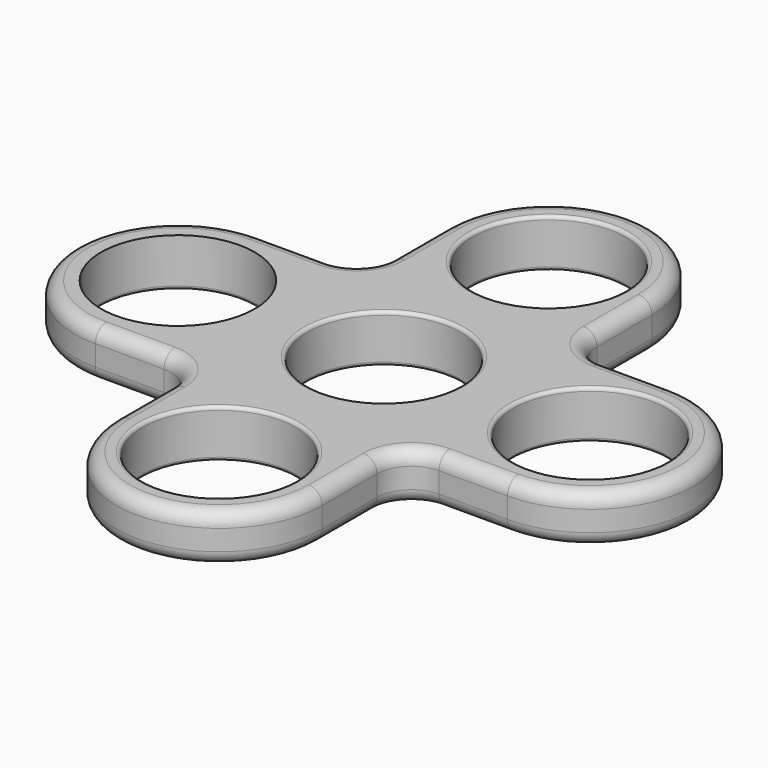
from build123d import *

# Parameters (mm, degrees)
F0_R     = 11.175
F1_DEPTH = 7
F2_R     = 5
F3_R     = 0.5
F4_R     = 2


# Not quite as in the source:
# - a feature names something its author has since deleted; it is built from what else it names


with BuildPart() as f1:
    # F0 (on Top) → F1 (new body)
    with BuildSketch(Plane.XY):
        with BuildLine():
            ThreePointArc((0.5794421554, 15.011195952), (10.8095243265, 19.6002796271), (15, 30))
            ThreePointArc((15, 30), (0, 45), (-15, 30))
            ThreePointArc((-15, 30), (-10.8095243265, 19.6002796271), (-0.5794421554, 15.011195952))
            Line((-0.5794421554, 15.011195952), (-0.011195952, 15.011195952))
            Line((-0.011195952, 15.011195952), (0.011195952, 15.011195952))
            Line((0.011195952, 15.011195952), (0.5794421554, 15.011195952))
        make_face()
        with Locations((0, 30)):
            Circle(F0_R, mode=Mode.SUBTRACT)
        with BuildLine():
            Line((15, 15.011195952), (15, 30))
            ThreePointArc((15, 30), (10.8095243265, 19.6002796271), (0.5794421554, 15.011195952))
            Line((0.5794421554, 15.011195952), (15, 15.011195952))
        make_face()
        with BuildLine():
            ThreePointArc((-0.5794421554, 15.011195952), (-10.8095243265, 19.6002796271), (-15, 30))
            Line((-15, 30), (-15, 15.011195952))
            Line((-15, 15.011195952), (-0.5794421554, 15.011195952))
        make_face()
        with BuildLine():
            Line((15, 15.011195952), (0.5794421554, 15.011195952))
            ThreePointArc((0.5794421554, 15.011195952), (0, 15), (-0.5794421554, 15.011195952))
            Line((-0.5794421554, 15.011195952), (-15, 15.011195952))
            Line((-15, 15.011195952), (-15, 0.5906381074))
            ThreePointArc((-15, 0.5906381074), (-14.9916032972, 0.3009711066), (-14.988804048, 0.011195952))
            ThreePointArc((-14.988804048, 0.011195952), (-14.9888050926, 0.0055979756), (-14.9888082263, 0))
            Line((-14.9888082263, 0), (-11.175, 0))
            ThreePointArc((-11.175, 0), (0, 11.175), (11.175, 0))
            Line((11.175, 0), (14.9888082263, 0))
            ThreePointArc((14.9888082263, 0), (14.9914961979, 0.2953741547), (15, 0.5906381074))
            Line((15, 0.5906381074), (15, 15.011195952))
        make_face()
        with BuildLine():
            ThreePointArc((-0.5794421554, 15.011195952), (0, 15), (0.5794421554, 15.011195952))
            Line((0.5794421554, 15.011195952), (0.011195952, 15.011195952))
            Line((0.011195952, 15.011195952), (-0.011195952, 15.011195952))
            Line((-0.011195952, 15.011195952), (-0.5794421554, 15.011195952))
        make_face()
        with BuildLine():
            Line((29.988804048, 15.011195952), (15, 15.011195952))
            Line((15, 15.011195952), (15, 0.5906381074))
            ThreePointArc((15, 0.5906381074), (19.5890836751, 10.8207202785), (29.988804048, 15.011195952))
        make_face()
        with BuildLine():
            Line((-15, 0.5906381074), (-15, 15.011195952))
            Line((-15, 15.011195952), (-29.988804048, 15.011195952))
            ThreePointArc((-29.988804048, 15.011195952), (-19.5890836751, 10.8207202785), (-15, 0.5906381074))
        make_face()
        with BuildLine():
            ThreePointArc((29.988804048, 15.011195952), (19.5890836751, 10.8207202785), (15, 0.5906381074))
            Line((15, 0.5906381074), (15, 0.0223919041))
            Line((15, 0.0223919041), (15, 0))
            Line((15, 0), (15, -0.5682462034))
            ThreePointArc((15, -0.5682462034), (19.5890836751, -10.7983283745), (29.988804048, -14.988804048))
            ThreePointArc((29.988804048, -14.988804048), (40.5954057658, -10.5954057658), (44.988804048, 0.011195952))
            ThreePointArc((44.988804048, 0.011195952), (40.5954057658, 10.6177976698), (29.988804048, 15.011195952))
        make_face()
        with Locations((29.988804048, 0.011195952)):
            Circle(F0_R, mode=Mode.SUBTRACT)
        with BuildLine():
            Line((15, 0.0223919041), (15, 0.5906381074))
            ThreePointArc((15, 0.5906381074), (14.9914961979, 0.2953741547), (14.9888082263, 0))
            Line((14.9888082263, 0), (15, 0))
            Line((15, 0), (15, 0.0223919041))
        make_face()
        with BuildLine():
            ThreePointArc((-14.988804048, 0.011195952), (-14.9916032972, 0.3009711066), (-15, 0.5906381074))
            Line((-15, 0.5906381074), (-15, 0.0223919041))
            Line((-15, 0.0223919041), (-15, 0))
            Line((-15, 0), (-14.9888082263, 0))
            ThreePointArc((-14.9888082263, 0), (-14.9888050926, 0.0055979756), (-14.988804048, 0.011195952))
        make_face()
        with BuildLine():
            Line((-15, 0.0223919041), (-15, 0.5906381074))
            ThreePointArc((-15, 0.5906381074), (-19.5890836751, 10.8207202785), (-29.988804048, 15.011195952))
            ThreePointArc((-29.988804048, 15.011195952), (-44.988804048, 0.011195952), (-29.988804048, -14.988804048))
            ThreePointArc((-29.988804048, -14.988804048), (-19.5890836751, -10.7983283745), (-15, -0.5682462034))
            Line((-15, -0.5682462034), (-15, 0))
            Line((-15, 0), (-15, 0.0223919041))
        make_face()
        with Locations((-29.988804048, 0.011195952)):
            Circle(F0_R, mode=Mode.SUBTRACT)
        with BuildLine():
            ThreePointArc((15, -0.5682462034), (14.9917124852, -0.2841761141), (14.9888082263, 0))
            Line((14.9888082263, 0), (11.175, 0))
            ThreePointArc((11.175, 0), (0, -11.175), (-11.175, 0))
            Line((-11.175, 0), (-14.9888082263, 0))
            ThreePointArc((-14.9888082263, 0), (-14.9917124852, -0.2841761141), (-15, -0.5682462034))
            Line((-15, -0.5682462034), (-15, -14.988804048))
            Line((-15, -14.988804048), (-0.5794421554, -14.988804048))
            ThreePointArc((-0.5794421554, -14.988804048), (0, -14.9776080959), (0.5794421554, -14.988804048))
            Line((0.5794421554, -14.988804048), (15, -14.988804048))
            Line((15, -14.988804048), (15, -0.5682462034))
        make_face()
        with BuildLine():
            Line((15, 0), (14.9888082263, 0))
            ThreePointArc((14.9888082263, 0), (14.9917124852, -0.2841761141), (15, -0.5682462034))
            Line((15, -0.5682462034), (15, 0))
        make_face()
        with BuildLine():
            ThreePointArc((-15, -0.5682462034), (-19.5890836751, -10.7983283745), (-29.988804048, -14.988804048))
            Line((-29.988804048, -14.988804048), (-15, -14.988804048))
            Line((-15, -14.988804048), (-15, -0.5682462034))
        make_face()
        with BuildLine():
            ThreePointArc((29.988804048, -14.988804048), (19.5890836751, -10.7983283745), (15, -0.5682462034))
            Line((15, -0.5682462034), (15, -14.988804048))
            Line((15, -14.988804048), (29.988804048, -14.988804048))
        make_face()
        with BuildLine():
            Line((-14.9888082263, 0), (-15, 0))
            Line((-15, 0), (-15, -0.5682462034))
            ThreePointArc((-15, -0.5682462034), (-14.9917124852, -0.2841761141), (-14.9888082263, 0))
        make_face()
        with BuildLine():
            Line((-0.5794421554, -14.988804048), (-15, -14.988804048))
            Line((-15, -14.988804048), (-15, -29.9776080959))
            ThreePointArc((-15, -29.9776080959), (-10.8095243265, -19.577887723), (-0.5794421554, -14.988804048))
        make_face()
        with BuildLine():
            Line((15, -29.9776080959), (15, -14.988804048))
            Line((15, -14.988804048), (0.5794421554, -14.988804048))
            ThreePointArc((0.5794421554, -14.988804048), (10.8095243265, -19.577887723), (15, -29.9776080959))
        make_face()
        with BuildLine():
            ThreePointArc((0.5794421554, -14.988804048), (0, -14.9776080959), (-0.5794421554, -14.988804048))
            Line((-0.5794421554, -14.988804048), (-0.011195952, -14.988804048))
            Line((-0.011195952, -14.988804048), (0.011195952, -14.988804048))
            Line((0.011195952, -14.988804048), (0.5794421554, -14.988804048))
        make_face()
        with BuildLine():
            Line((-0.011195952, -14.988804048), (-0.5794421554, -14.988804048))
            ThreePointArc((-0.5794421554, -14.988804048), (-10.8095243265, -19.577887723), (-15, -29.9776080959))
            ThreePointArc((-15, -29.9776080959), (0, -44.9776080959), (15, -29.9776080959))
            ThreePointArc((15, -29.9776080959), (10.8095243265, -19.577887723), (0.5794421554, -14.988804048))
            Line((0.5794421554, -14.988804048), (0.011195952, -14.988804048))
            Line((0.011195952, -14.988804048), (-0.011195952, -14.988804048))
        make_face()
        with Locations((0, -29.9776080959)):
            Circle(F0_R, mode=Mode.SUBTRACT)
    extrude(amount=F1_DEPTH)

    # F2
    f2_edges = [f1.edges().sort_by_distance(p)[0] for p in [
        (-15, 30, 3.5),
        (-15, 15.011196, 3.5),
        (15, 30, 3.5),
        (15, 15.011196, 3.5),
        (15, -14.988804, 3.5),
        (-15, -14.988804, 3.5),
    ]]
    fillet(f2_edges, radius=F2_R)

    # F3
    f3_edges = [f1.edges().sort_by_distance(p)[0] for p in [
        (-11.175, 30, 7),
        (-11.175, 0, 7),
        (-11.175, 30, 0),
        (-11.175, 0, 0),
        (-11.175, -29.977608, 7),
        (-41.163804, 0.011196, 0),
        (18.813804, 0.011196, 0),
        (-11.175, -29.977608, 0),
        (18.813804, 0.011196, 7),
    ]]
    fillet(f3_edges, radius=F3_R)

    # F4
    f4_edges = [f1.edges().sort_by_distance(p)[0] for p in [
        (-16.464466, 16.475662, 0),
        (-15, 20.011196, 3.5),
        (-20, 15.011196, 3.5),
        (-16.464466, 16.475662, 7),
        (-15, 25.005598, 0),
        (-15, 30, 3.5),
        (-15, 25.005598, 7),
        (15, 30, 3.5),
        (0, 45, 0),
        (0, 45, 7),
        (15, 25.005598, 0),
        (15, 20.011196, 3.5),
        (15, 25.005598, 7),
        (16.464466, 16.475662, 0),
        (20, 15.011196, 3.5),
        (16.464466, 16.475662, 7),
        (0, -44.977608, 7),
        (0, -44.977608, 0),
        (-24.994402, -14.988804, 0),
        (-16.464466, -16.45327, 0),
        (-44.988804, 0.011196, 0),
        (-15, -24.983206, 0),
        (-24.994402, 15.011196, 0),
        (15, -24.983206, 0),
        (16.464466, -16.45327, 0),
        (24.994402, -14.988804, 0),
        (44.988804, 0.011196, 0),
        (24.994402, 15.011196, 0),
        (-24.994402, -14.988804, 7),
        (-16.464466, -16.45327, 7),
        (-44.988804, 0.011196, 7),
        (-15, -24.983206, 7),
        (-24.994402, 15.011196, 7),
        (15, -24.983206, 7),
        (16.464466, -16.45327, 7),
        (24.994402, -14.988804, 7),
        (44.988804, 0.011196, 7),
        (24.994402, 15.011196, 7),
    ]]
    fillet(f4_edges, radius=F4_R)


solid = f1.part
